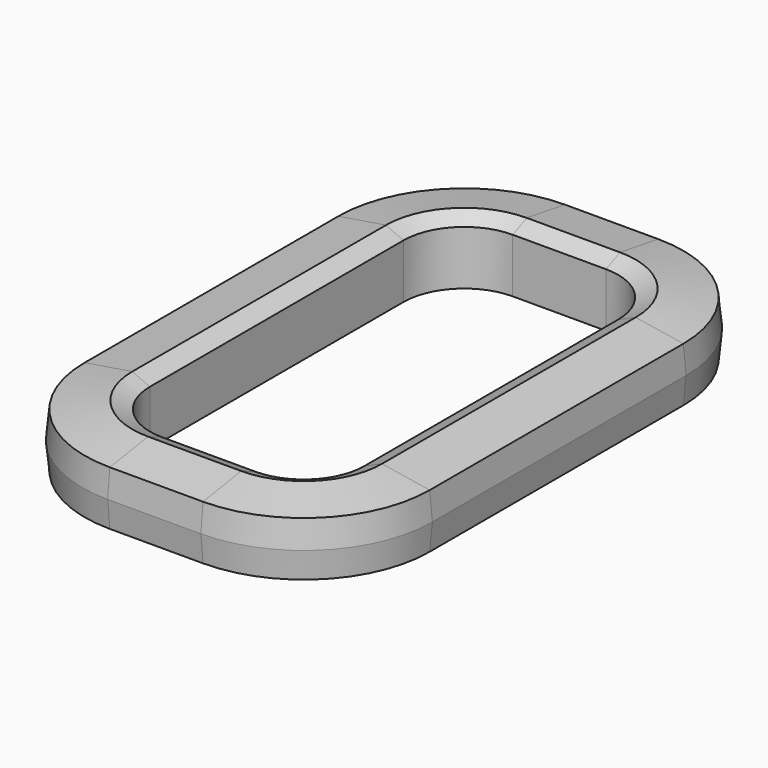
from build123d import *


# Not quite as in the source:
# - a feature names something its author has since deleted; it is built from what else it names


with BuildPart() as f2:
    # F2: sweep along a path in F0
    with BuildLine(Plane.XY) as f2_path:
        Line((-7.5, -8.5), (-7.5, 8.5))
        ThreePointArc((-7.5, 8.5), (-6.0355339059, 12.0355339059), (-2.5, 13.5))
        Line((-2.5, 13.5), (2.5, 13.5))
        ThreePointArc((2.5, 13.5), (6.0355339059, 12.0355339059), (7.5, 8.5))
        Line((7.5, 8.5), (7.5, -8.5))
        ThreePointArc((7.5, -8.5), (6.0355339059, -12.0355339059), (2.5, -13.5))
        Line((2.5, -13.5), (-2.5, -13.5))
        ThreePointArc((-2.5, -13.5), (-6.0355339059, -12.0355339059), (-7.5, -8.5))
    # F1 (on Front) → F2 (sweep)
    with BuildSketch(Plane.XZ):
        Polygon((-5.751425866, 1.454347861), (-6.6942584633, 1.8659339551), (-9.2492606491, 1.454347861), (-9.3934396282, 0), (-9.2492606491, -1.454347861), (-6.6942584633, -1.8659339551), (-5.751425866, -1.454347861), (-5.751425866, 0), align=None)
    sweep(path=f2_path.line)


solid = f2.part
